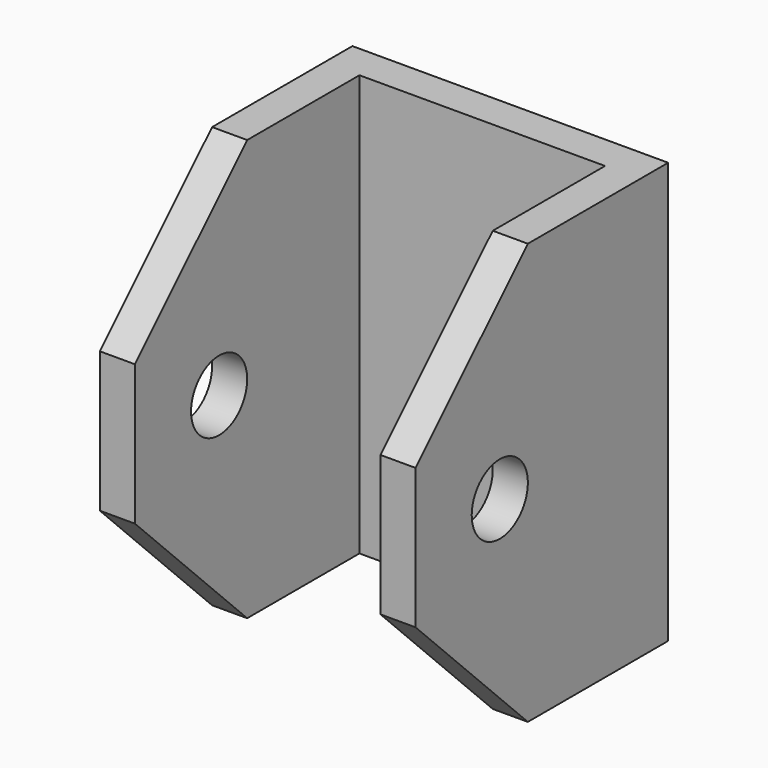
from build123d import *

# Parameters (mm, degrees)
F0_W      = 45
F0_H      = 60
F1_DEPTH  = 5
F2_W      = 5
F2_H      = 60
F3_DEPTH  = 40
F4_SIZE2  = 20
F4_SIZE   = 20
F5_R      = 5
F6_DEPTH  = 50
F8_D      = 6
F8_DEPTH  = 20
F8_TIP    = 1.8025818571
F10_DEPTH = 2
F11_DEPTH = 2


# Not quite as in the source:
# - after a boolean that leaves OpenCascade's solid faulty, fix() repairs it


with BuildPart() as f1:
    # F0 (on Front) → F1 (new body)
    with BuildSketch(Plane.XZ):
        Rectangle(F0_W, F0_H)
    extrude(amount=F1_DEPTH)

    # F2 (on face) → F3 (join)
    with BuildSketch(Plane.XZ.offset(5)):
        with Locations((-20, 0)):
            Rectangle(F2_W, F2_H)
        with Locations((20, 0)):
            Rectangle(F2_W, F2_H)
    extrude(amount=F3_DEPTH)

    # F4
    f4_edges = [f1.edges().sort_by_distance(p)[0] for p in [
        (20, -45, 30),
        (-20, -45, 30),
        (20, -45, -30),
        (-20, -45, -30),
    ]]
    chamfer(f4_edges, length=F4_SIZE, length2=F4_SIZE2)

    # F5 (on face) → F6 (cut)
    with BuildSketch(Plane(origin=(-22.5, 0, 0), x_dir=(0, -1, 0), z_dir=(-1, 0, 0))):
        with Locations((30, 0)):
            Circle(F5_R)
    extrude(amount=-F6_DEPTH, mode=Mode.SUBTRACT)

    # F8
    with Locations(Plane.XZ.offset(5)):
        with Locations((0, 0)):
            Hole(F8_D / 2, depth=F8_DEPTH)
            with Locations((0, 0, -(F8_DEPTH + F8_TIP / 2))):  # 118° drill point
                Cone(0, F8_D / 2, F8_TIP, mode=Mode.SUBTRACT)

    # F9 (on face) → F10 (cut)
    with BuildSketch(Plane(origin=(0, 0, 0), x_dir=(-1, 0, 0), z_dir=(0, 1, 0))):
        with BuildLine():
            Line((-5, -1), (-3.7431358354, -1))
            ThreePointArc((-3.7431358354, -1), (-3.8701524892, 0), (-3.7431358354, 1))
            Line((-3.7431358354, 1), (-5, 1))
            Line((-5, 1), (-5, -1))
        make_face()
        with BuildLine():
            ThreePointArc((-1, 3.8371140982), (-0.0042634526, 3.997751149), (1, 3.9042073005))
            Line((1, 3.9042073005), (1, 5))
            Line((1, 5), (-1, 5))
            Line((-1, 5), (-1, 3.8371140982))
        make_face()
        with BuildLine():
            Line((4.002830857, -1), (5, -1))
            Line((5, -1), (5, 1))
            Line((5, 1), (4.002830857, 1))
            ThreePointArc((4.002830857, 1), (4.0979662959, 0.5040171699), (4.1298475108, 0))
            ThreePointArc((4.1298475108, 0), (4.0979662959, -0.5040171699), (4.002830857, -1))
        make_face()
        with BuildLine():
            Line((1, -5), (1, -3.9042073005))
            ThreePointArc((1, -3.9042073005), (-0.0042634526, -3.997751149), (-1, -3.8371140982))
            Line((-1, -3.8371140982), (-1, -5))
            Line((-1, -5), (1, -5))
        make_face()
    extrude(amount=-F10_DEPTH, mode=Mode.SUBTRACT)

    # F9 (on face) → F11 (cut)
    with BuildSketch(Plane(origin=(0, 0, 0), x_dir=(-1, 0, 0), z_dir=(0, 1, 0))):
        with BuildLine():
            Line((2.8284271247, -1), (4.002830857, -1))
            ThreePointArc((4.002830857, -1), (4.0979662959, -0.5040171699), (4.1298475108, 0))
            ThreePointArc((4.1298475108, 0), (4.0979662959, 0.5040171699), (4.002830857, 1))
            Line((4.002830857, 1), (2.8284271247, 1))
            ThreePointArc((2.8284271247, 1), (2.956795679, 0.5073059362), (3, 0))
            ThreePointArc((3, 0), (2.956795679, -0.5073059362), (2.8284271247, -1))
        make_face()
        with BuildLine():
            ThreePointArc((-3.7431358354, 1), (-3.8701524892, 0), (-3.7431358354, -1))
            Line((-3.7431358354, -1), (-2.8284271247, -1))
            ThreePointArc((-2.8284271247, -1), (-3, 0), (-2.8284271247, 1))
            Line((-2.8284271247, 1), (-3.7431358354, 1))
        make_face()
        with BuildLine():
            Line((1, 2.8284271247), (1, 3.9042073005))
            ThreePointArc((1, 3.9042073005), (-0.0042634526, 3.997751149), (-1, 3.8371140982))
            Line((-1, 3.8371140982), (-1, 2.8284271247))
            ThreePointArc((-1, 2.8284271247), (0, 3), (1, 2.8284271247))
        make_face()
        with BuildLine():
            ThreePointArc((-1, -3.8371140982), (-0.0042634526, -3.997751149), (1, -3.9042073005))
            Line((1, -3.9042073005), (1, -2.8284271247))
            ThreePointArc((1, -2.8284271247), (0, -3), (-1, -2.8284271247))
            Line((-1, -2.8284271247), (-1, -3.8371140982))
        make_face()
    extrude(amount=-F11_DEPTH, mode=Mode.SUBTRACT)

    add(f1.part.fix(), mode=Mode.REPLACE)


solid = f1.part
